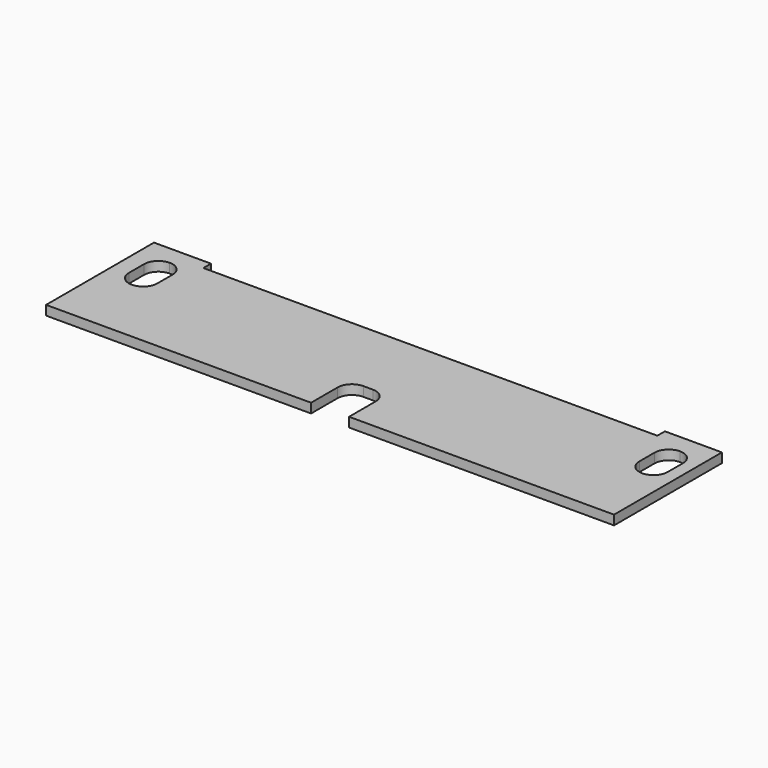
from build123d import *

# Parameters (mm, degrees)
F0_W     = 3
F0_H     = 5
F1_DEPTH = 1
F2_R     = 1.49999
F3_R     = 1.5


# Not quite as in the source:
# - a fillet or chamfer is up to 0.001 mm smaller than in the source, because OpenCascade refuses the exact size


with BuildPart() as f1:
    # F0 (on Top) → F1 (new body)
    with BuildSketch(Plane.XY):
        Polygon((-13.5924067289, 6.5421499412), (-19.5924067289, 6.5421499412), (-19.5924067289, -7.6578500588), (8.3075932711, -7.6578500588), (8.3075932711, -2.6578500588), (12.3075932711, -2.6578500588), (12.3075932711, -7.6578500588), (40.2075932711, -7.6578500588), (40.2075932711, 6.5421499412), (34.2075932711, 6.5421499412), (34.2075932711, 5.5421499412), (-13.5924067289, 5.5421499412), align=None)
        with Locations((-16.332133919, 2.0421499412)):
            Rectangle(F0_W, F0_H, mode=Mode.SUBTRACT)
        with Locations((37.4102636576, 2.0421499412)):
            Rectangle(F0_W, F0_H, mode=Mode.SUBTRACT)
    extrude(amount=F1_DEPTH)

    # F2 (radius 1.5 in the source; OpenCascade refuses exactly that, so slightly less here)
    f2_edges = [f1.edges().sort_by_distance(p)[0] for p in [
        (-17.832134, 4.54215, 0.5),
        (-14.832134, 4.54215, 0.5),
        (-14.832134, -0.45785, 0.5),
        (-17.832134, -0.45785, 0.5),
        (38.910264, 4.54215, 0.5),
        (35.910264, 4.54215, 0.5),
        (35.910264, -0.45785, 0.5),
        (38.910264, -0.45785, 0.5),
    ]]
    fillet(f2_edges, radius=F2_R)

    # F3
    f3_edges = [f1.edges().sort_by_distance(p)[0] for p in [
        (8.307593, -2.65785, 0.5),
        (12.307593, -2.65785, 0.5),
    ]]
    fillet(f3_edges, radius=F3_R)


solid = f1.part
